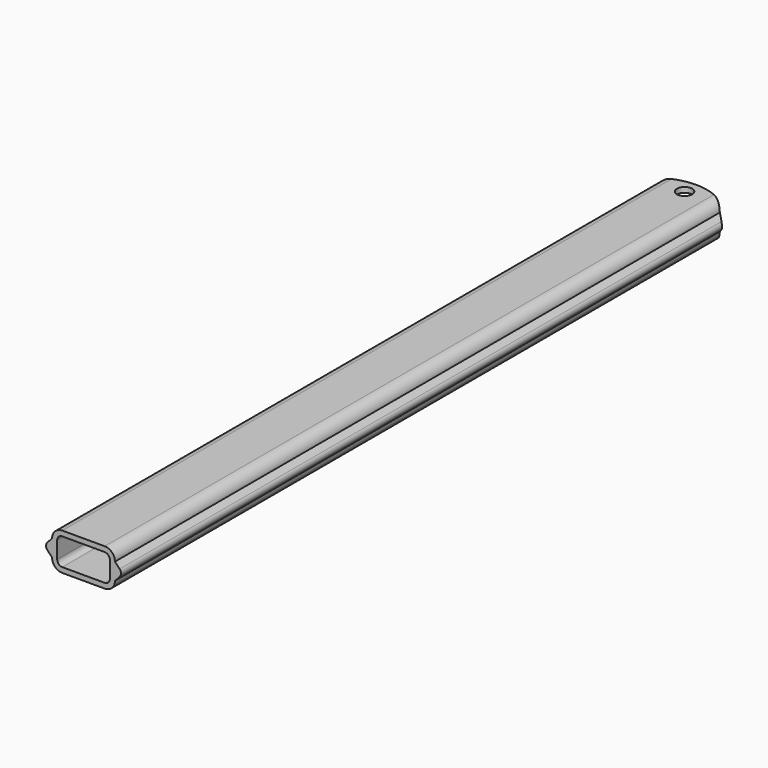
from build123d import *

# Parameters (mm, degrees)
F1_DEPTH = 150
F2_R     = 1.5
F3_DEPTH = 7.301
F6_DEPTH = 25


# Not quite as in the source:
# - a feature names something its author has since deleted; it is built from what else it names


with BuildPart() as f1:
    # F0 (on Front) → F1 (new body)
    with BuildSketch(Plane.XZ):
        with BuildLine():
            Line((7.0581561667, 0.685534298), (6.15, 1.65))
            ThreePointArc((6.15, 1.65), (5.5642135624, 3.0642135624), (4.15, 3.65))
            Line((4.15, 3.65), (-4.15, 3.65))
            ThreePointArc((-4.15, 3.65), (-5.5642135624, 3.0642135624), (-6.15, 1.65))
            Line((-6.15, 1.65), (-7.0581561667, 0.685534298))
            ThreePointArc((-7.0581561667, 0.685534298), (-7.3301158338, 0), (-7.0581561667, -0.685534298))
            Line((-7.0581561667, -0.685534298), (-6.15, -1.65))
            ThreePointArc((-6.15, -1.65), (-5.5642135624, -3.0642135624), (-4.15, -3.65))
            Line((-4.15, -3.65), (4.15, -3.65))
            ThreePointArc((4.15, -3.65), (5.5642135624, -3.0642135624), (6.15, -1.65))
            Line((6.15, -1.65), (7.0581561667, -0.685534298))
            ThreePointArc((7.0581561667, -0.685534298), (7.3301158338, 0), (7.0581561667, 0.685534298))
        make_face()
        with BuildLine():
            ThreePointArc((5.15, -1.65), (4.8571067812, -2.3571067812), (4.15, -2.65))
            Line((4.15, -2.65), (-4.15, -2.65))
            ThreePointArc((-4.15, -2.65), (-4.8571067812, -2.3571067812), (-5.15, -1.65))
            Line((-5.15, -1.65), (-5.15, 1.65))
            ThreePointArc((-5.15, 1.65), (-4.8571067812, 2.3571067812), (-4.15, 2.65))
            Line((-4.15, 2.65), (4.15, 2.65))
            ThreePointArc((4.15, 2.65), (4.8571067812, 2.3571067812), (5.15, 1.65))
            Line((5.15, 1.65), (5.15, -1.65))
        make_face(mode=Mode.SUBTRACT)
    extrude(amount=F1_DEPTH)

    # F2 (on face) → F3 (cut, through all)
    with BuildSketch(Plane.XY.offset(3.65)):
        with Locations((0, -3)):
            Circle(F2_R)
    extrude(amount=-F3_DEPTH, mode=Mode.SUBTRACT)

    # F5 (on offset) → F6 (cut)
    with BuildSketch(Plane.XY.offset(4.6)):
        with BuildLine():
            Line((8, -3.7011680724), (8, 3.7011680724))
            Line((8, 3.7011680724), (-8, 3.7011680724))
            Line((-8, 3.7011680724), (-8, -3.7011680724))
            ThreePointArc((-8, -3.7011680724), (0, -0.1482238292), (8, -3.7011680724))
        make_face()
    extrude(amount=-F6_DEPTH, mode=Mode.SUBTRACT)


solid = f1.part
